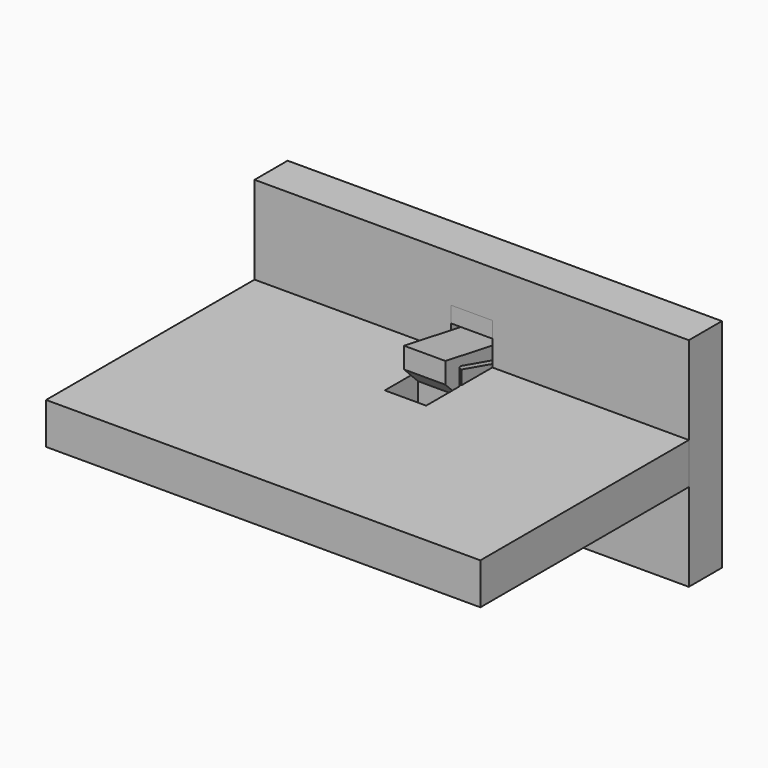
from build123d import *

# Parameters (mm, degrees)
F2_DEPTH = 2.38125
F3_W     = 50
F3_H     = 25
F3_W_2   = 4.7625
F3_H_2   = 14.2875
F4_DEPTH = 4.7625
F6_DEPTH = 2.38125


# Not quite as in the source:
# - a length typed as a fraction of an inch, garbled in the dataset ("3 / 203.2 mm" for 3/8 in), is restored


with BuildPart() as f2:
    # F1 (on Top) → F2 (new body, symmetric)
    with BuildSketch(Plane.XY):
        Polygon((-2.38125, 0), (-25, 0), (-25, -30), (0, -30), (25, -30), (25, 0), (2.38125, 0), (2.38125, -2.38125), (0, -2.38125), (-2.38125, -2.38125), align=None)
        Polygon((-2.38125, -4.7625), (0, -4.7625), (2.38125, -4.7625), (2.38125, -9.525), (0, -9.525), (-2.38125, -9.525), align=None, mode=Mode.SUBTRACT)
    extrude(amount=F2_DEPTH, both=True)


with BuildPart() as f4:
    # F3 (on Front) → F4 (new body)
    with BuildSketch(Plane.XZ):
        Rectangle(F3_W, F3_H)
        Rectangle(F3_W_2, F3_H_2, mode=Mode.SUBTRACT)
    extrude(amount=-F4_DEPTH)


with BuildPart() as f6:
    # F5 (on Right) → F6 (new body, symmetric)
    with BuildSketch(Plane.YZ):
        with BuildLine():
            Line((4.7625, 9.525), (4.7625, 7.14375))
            Line((4.7625, 7.14375), (0, 7.14375))
            Line((0, 7.14375), (0, 5.3015985947))
            Line((0, 5.3015985947), (4.8354205115, 4.1182366897))
            ThreePointArc((4.8354205115, 4.1182366897), (4.9671724392, 3.9090526811), (4.7625, 3.7703958653))
            Line((4.7625, 3.7703958653), (-6.7625, 5.7876744365))
            Line((-6.7625, 5.7876744365), (-6.7625, 3.38125))
            Line((-6.7625, 3.38125), (-4.7625, 1.38125))
            Line((-4.7625, 1.38125), (-4.7625, 2.38125))
            Line((-4.7625, 2.38125), (-4.7625, 4.2031772012))
            ThreePointArc((-4.7625, 4.2031772012), (-4.6921440652, 4.3448409329), (-4.5367563233, 4.3743912306))
            Line((-4.5367563233, 4.3743912306), (4.7625, 1.7703958653))
            ThreePointArc((4.7625, 1.7703958653), (4.8857703527, 1.5512381592), (4.6666126465, 1.4279678065))
            Line((4.6666126465, 1.4279678065), (-4.4069, 3.96875))
            Line((-4.4069, 3.96875), (-4.4069, 2.38125))
            Line((-4.4069, 2.38125), (-2.38125, 2.38125))
            Line((-2.38125, 2.38125), (-2.38125, 0))
            Line((-2.38125, 0), (-2.38125, -2.38125))
            Line((-2.38125, -2.38125), (-4.4069, -2.38125))
            Line((-4.4069, -2.38125), (-4.4069, -3.96875))
            Line((-4.4069, -3.96875), (4.6666126465, -1.4279678065))
            ThreePointArc((4.6666126465, -1.4279678065), (4.8857703527, -1.5512381592), (4.7625, -1.7703958653))
            Line((4.7625, -1.7703958653), (-4.5367563233, -4.3743912306))
            ThreePointArc((-4.5367563233, -4.3743912306), (-4.6921440652, -4.3448409329), (-4.7625, -4.2031772012))
            Line((-4.7625, -4.2031772012), (-4.7625, -2.38125))
            Line((-4.7625, -2.38125), (-4.7625, -1.38125))
            Line((-4.7625, -1.38125), (-6.7625, -3.38125))
            Line((-6.7625, -3.38125), (-6.7625, -5.7876744365))
            Line((-6.7625, -5.7876744365), (4.7625, -3.7703958653))
            ThreePointArc((4.7625, -3.7703958653), (4.9671724392, -3.9090526811), (4.8354205115, -4.1182366897))
            Line((4.8354205115, -4.1182366897), (0, -5.3015985947))
            Line((0, -5.3015985947), (0, -7.14375))
            Line((0, -7.14375), (4.7625, -7.14375))
            Line((4.7625, -7.14375), (4.7625, -9.525))
            Line((4.7625, -9.525), (7.14375, -9.525))
            Line((7.14375, -9.525), (7.14375, 0))
            Line((7.14375, 0), (7.14375, 9.525))
            Line((7.14375, 9.525), (4.7625, 9.525))
        make_face()
    extrude(amount=F6_DEPTH, both=True)


solid = Compound([f2.part, f4.part, f6.part])
